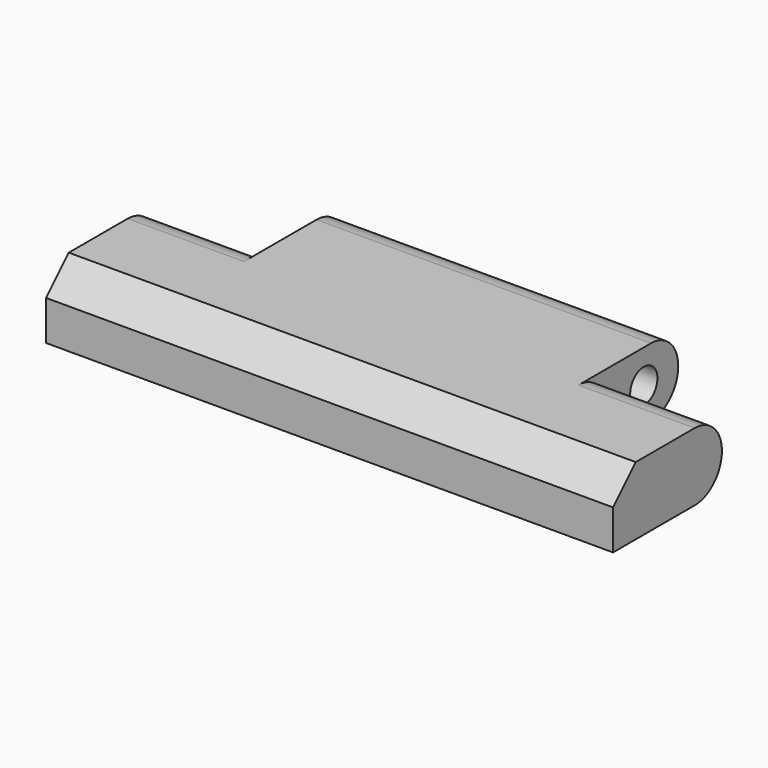
from build123d import *

# Parameters (mm, degrees)
F1_DEPTH = 6
F2_R     = 2.99999
F3_R     = 1.5
F4_DEPTH = 39.751
F5_SIZE  = 2.5


# Not quite as in the source:
# - a fillet or chamfer is up to 0.001 mm smaller than in the source, because OpenCascade refuses the exact size


with BuildPart() as f1:
    # F0 (on Top) → F1 (new body)
    with BuildSketch(Plane.XY):
        Polygon((0, -5.7625164015), (0, -17.7625164015), (50, -17.7625164015), (50, -5.7625164015), (39.75, -5.7625164015), (39.75, 2.2374835985), (10.25, 2.2374835985), (10.25, -5.7625164015), align=None)
    extrude(amount=F1_DEPTH)

    # F2 (radius 3 in the source; OpenCascade refuses exactly that, so slightly less here)
    f2_edges = [f1.edges().sort_by_distance(p)[0] for p in [
        (25, 2.237484, 6),
        (25, 2.237484, 0),
        (5.125, -5.762516, 6),
        (44.875, -5.762516, 6),
        (5.125, -5.762516, 0),
        (44.875, -5.762516, 0),
    ]]
    fillet(f2_edges, radius=F2_R)

    # F3 (on face) → F4 (cut, through all)
    with BuildSketch(Plane(origin=(10.25, 0, 0), x_dir=(0, -1, 0), z_dir=(-1, 0, 0))):
        with Locations((1.5625164015, 3)):
            Circle(F3_R)
    extrude(amount=-F4_DEPTH, mode=Mode.SUBTRACT)

    # F5
    f5_edges = [f1.edges().sort_by_distance(p)[0] for p in [
        (25, -17.762516, 6),
    ]]
    chamfer(f5_edges, length=F5_SIZE)


solid = f1.part
